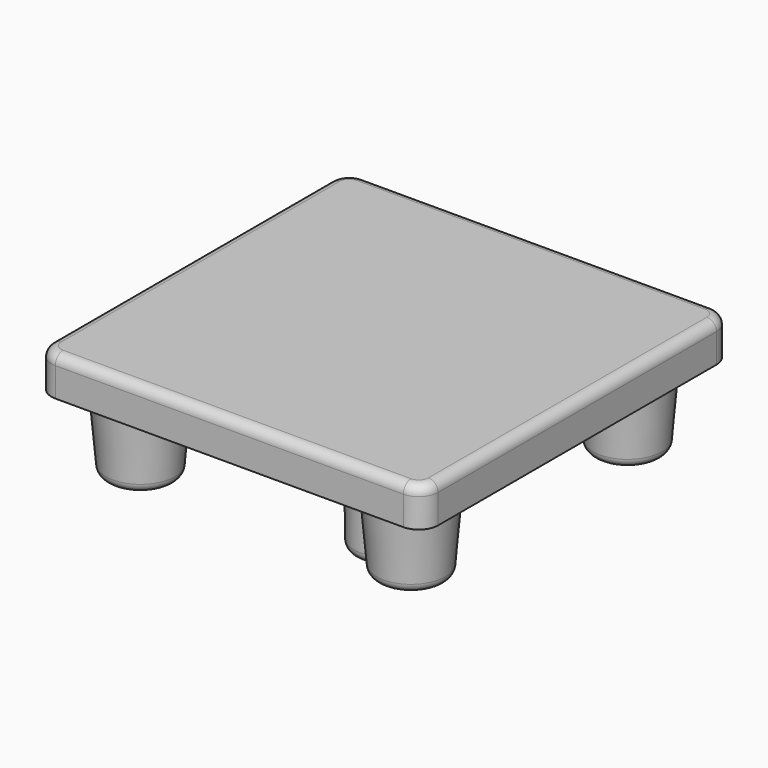
from build123d import *

# Parameters (mm, degrees)
F0_W                     = 20
F0_H                     = 20
F0_R                     = 2.1
F1_DEPTH                 = 2
F2_DEPTH                 = 4
F2_TAPER                 = 5
F3_DEPTH                 = 8
DRAFT_F3_DRAFTED_ANGLE   = 1
DRAFT_F3_2_DRAFTED_ANGLE = 1
F4_R                     = 1
F5_T12_ANGLE             = 249.4018409202
F5_T17_ANGLE             = 249.4018409202
F5_T19_DEPTH             = 18
F5_T21_DEPTH             = 18
F5_T24_ANGLE             = 90
F5_T26_ANGLE             = 90
F5_T28_ANGLE             = 90
F5_T30_ANGLE             = 90
F5_T42_ANGLE             = 245.17376067
F5_T47_ANGLE             = 245.17376067


# Not quite as in the source:
# - a fillet or chamfer that OpenCascade refuses, or shapes differently, is made with other operations: its cross-section is extruded or revolved along the edge and cut away or added
# - an extrude with a draft is written as a straight extrude whose walls are then drafted


with BuildPart() as f1:
    # F0 (on Top) → F1 (new body)
    with BuildSketch(Plane.XY):
        with Locations((-49.5571177453, 39.7264205217)):
            Rectangle(F0_W, F0_H)
        with Locations((-56.5571177453, 32.7264205217)):
            Circle(F0_R, mode=Mode.SUBTRACT)
        with BuildLine():
            ThreePointArc((-47.8689234437, 39.9264205217), (-47.8600717364, 39.8265945884), (-47.8571177453, 39.7264205217))
            ThreePointArc((-47.8571177453, 39.7264205217), (-47.8600717364, 39.6262464551), (-47.8689234437, 39.5264205217))
            ThreePointArc((-47.8689234437, 39.5264205217), (-49.5571177453, 38.0264205217), (-51.2453120469, 39.5264205217))
            ThreePointArc((-51.2453120469, 39.5264205217), (-51.2571177453, 39.7264205217), (-51.2453120469, 39.9264205217))
            ThreePointArc((-51.2453120469, 39.9264205217), (-49.5571177453, 41.4264205217), (-47.8689234437, 39.9264205217))
        make_face(mode=Mode.SUBTRACT)
        with Locations((-42.5571177453, 32.7264205217)):
            Circle(F0_R, mode=Mode.SUBTRACT)
        with Locations((-56.5571177453, 46.7264205217)):
            Circle(F0_R, mode=Mode.SUBTRACT)
        with Locations((-42.5571177453, 46.7264205217)):
            Circle(F0_R, mode=Mode.SUBTRACT)
        with Locations((-42.5571177453, 46.7264205217)):
            Circle(F0_R)
        with Locations((-42.5571177453, 32.7264205217)):
            Circle(F0_R)
        with Locations((-56.5571177453, 32.7264205217)):
            Circle(F0_R)
        with Locations((-56.5571177453, 46.7264205217)):
            Circle(F0_R)
        with BuildLine():
            ThreePointArc((-47.8689234437, 39.5264205217), (-47.8600717364, 39.6262464551), (-47.8571177453, 39.7264205217))
            ThreePointArc((-47.8571177453, 39.7264205217), (-47.8600717364, 39.8265945884), (-47.8689234437, 39.9264205217))
            Line((-47.8689234437, 39.9264205217), (-51.2453120469, 39.9264205217))
            ThreePointArc((-51.2453120469, 39.9264205217), (-51.2571177453, 39.7264205217), (-51.2453120469, 39.5264205217))
            Line((-51.2453120469, 39.5264205217), (-47.8689234437, 39.5264205217))
        make_face()
        with BuildLine():
            Line((-51.2453120469, 39.9264205217), (-47.8689234437, 39.9264205217))
            ThreePointArc((-47.8689234437, 39.9264205217), (-49.5571177453, 41.4264205217), (-51.2453120469, 39.9264205217))
        make_face()
        with BuildLine():
            ThreePointArc((-51.2453120469, 39.5264205217), (-49.5571177453, 38.0264205217), (-47.8689234437, 39.5264205217))
            Line((-47.8689234437, 39.5264205217), (-51.2453120469, 39.5264205217))
        make_face()
    extrude(amount=F1_DEPTH)

    # F0 (on Top) → F2 (join)
    with BuildSketch(Plane.XY):
        with Locations((-42.5571177453, 46.7264205217)):
            Circle(F0_R)
        with Locations((-56.5571177453, 46.7264205217)):
            Circle(F0_R)
        with Locations((-56.5571177453, 32.7264205217)):
            Circle(F0_R)
        with Locations((-42.5571177453, 32.7264205217)):
            Circle(F0_R)
    extrude(amount=-F2_DEPTH, taper=F2_TAPER)


with BuildPart() as f3_drafted:
    # F0 (on Top) → F3 (new body)
    with BuildSketch(Plane.XY):
        with BuildLine():
            Line((-51.2453120469, 39.9264205217), (-47.8689234437, 39.9264205217))
            ThreePointArc((-47.8689234437, 39.9264205217), (-49.5571177453, 41.4264205217), (-51.2453120469, 39.9264205217))
        make_face()
    extrude(amount=-F3_DEPTH)

    # draft_F3_drafted
    draft_f3_drafted_walls = [f3_drafted.faces().sort_by_distance(p)[0] for p in [
        (-49.5571177453, 39.9264205217, -5.3333333333),
        (-49.5571177453, 41.4264205217, -5.3333333333),
    ]]
    draft(draft_f3_drafted_walls, neutral_plane=Plane(origin=(0, 0, 0), x_dir=(1, 0, 0), z_dir=(0, 0, -1)), angle=DRAFT_F3_DRAFTED_ANGLE)


with BuildPart() as f1_1:
    add(f1.part)

    # join_F3_drafted: union F3_drafted
    add(f3_drafted.part)


with BuildPart() as f3_2_drafted:
    # F0 (on Top) → F3, piece 2 (new body)
    with BuildSketch(Plane.XY):
        with BuildLine():
            ThreePointArc((-51.2453120469, 39.5264205217), (-49.5571177453, 38.0264205217), (-47.8689234437, 39.5264205217))
            Line((-47.8689234437, 39.5264205217), (-51.2453120469, 39.5264205217))
        make_face()
    extrude(amount=-F3_DEPTH)

    # draft_F3_2_drafted
    draft_f3_2_drafted_walls = [f3_2_drafted.faces().sort_by_distance(p)[0] for p in [
        (-49.5571177453, 38.0264205217, -5.3333333333),
        (-49.5571177453, 39.5264205217, -5.3333333333),
    ]]
    draft(draft_f3_2_drafted_walls, neutral_plane=Plane(origin=(0, 0, 0), x_dir=(1, 0, 0), z_dir=(0, 0, -1)), angle=DRAFT_F3_2_DRAFTED_ANGLE)


with BuildPart() as f1_2:
    add(f1_1.part)

    # join_F3_2_drafted: union F3_2_drafted
    add(f3_2_drafted.part)

    # F4
    f4_edges = [f1_2.edges().sort_by_distance(p)[0] for p in [
        (-39.557118, 49.726421, 1),
        (-39.557118, 29.726421, 1),
        (-59.557118, 49.726421, 1),
        (-59.557118, 29.726421, 1),
    ]]
    fillet(f4_edges, radius=F4_R)

    # F5: fillet of radius 0.5 on 20 edges, made by hand

    # F5_s1 → F5_t2 (revolve)
    with BuildSketch(Plane.XZ.offset(-46.7264205217)):
        with BuildLine():
            ThreePointArc((-39.9989521583, 0), (-40.3367472621, -0.1313613316), (-40.4970495073, -0.4564221286))
            Line((-40.4970495073, -0.4564221286), (-40.5070114543, -0.4555505712))
            Line((-40.5070114543, -0.4555505712), (-40.466281057, 0.01))
            Line((-40.466281057, 0.01), (-39.9989521583, 0.01))
            Line((-39.9989521583, 0.01), (-39.9989521583, 0))
        make_face()
    revolve(axis=Axis((-42.5571177453, 46.7264205217, 0), (0, 0, -1)))

    # F5_s3 → F5_t4 (revolve)
    with BuildSketch(Plane.XZ.offset(-32.7264205217)):
        with BuildLine():
            ThreePointArc((-39.9989521583, 0), (-40.3367472621, -0.1313613316), (-40.4970495073, -0.4564221286))
            Line((-40.4970495073, -0.4564221286), (-40.5070114543, -0.4555505712))
            Line((-40.5070114543, -0.4555505712), (-40.466281057, 0.01))
            Line((-40.466281057, 0.01), (-39.9989521583, 0.01))
            Line((-39.9989521583, 0.01), (-39.9989521583, 0))
        make_face()
    revolve(axis=Axis((-42.5571177453, 32.7264205217, 0), (0, 0, -1)))

    # F5_s5 → F5_t6 (revolve)
    with BuildSketch(Plane.XZ.offset(-32.7264205217)):
        with BuildLine():
            ThreePointArc((-53.9989521583, 0), (-54.3367472621, -0.1313613316), (-54.4970495073, -0.4564221286))
            Line((-54.4970495073, -0.4564221286), (-54.5070114543, -0.4555505712))
            Line((-54.5070114543, -0.4555505712), (-54.466281057, 0.01))
            Line((-54.466281057, 0.01), (-53.9989521583, 0.01))
            Line((-53.9989521583, 0.01), (-53.9989521583, 0))
        make_face()
    revolve(axis=Axis((-56.5571177453, 32.7264205217, 0), (0, 0, -1)))

    # F5_s7 → F5_t8 (revolve)
    with BuildSketch(Plane.XZ.offset(-46.7264205217)):
        with BuildLine():
            ThreePointArc((-53.9989521583, 0), (-54.3367472621, -0.1313613316), (-54.4970495073, -0.4564221286))
            Line((-54.4970495073, -0.4564221286), (-54.5070114543, -0.4555505712))
            Line((-54.5070114543, -0.4555505712), (-54.466281057, 0.01))
            Line((-54.466281057, 0.01), (-53.9989521583, 0.01))
            Line((-53.9989521583, 0.01), (-53.9989521583, 0))
        make_face()
    revolve(axis=Axis((-56.5571177453, 46.7264205217, 0), (0, 0, -1)))


with BuildPart() as f5_tool10:
    # F5_s11 → F5_t12 (revolve)
    with BuildSketch(Plane(origin=(2.5321968025, 3.6568310809, 0), x_dir=(0, 0, 1), z_dir=(0.5692927311, 0.8221348954, 0))):
        with BuildLine():
            ThreePointArc((0, -65.5499468838), (-0.1433747754, -65.1994922516), (-0.4912737968, -65.0500230362))
            Line((-0.4912737968, -65.0500230362), (-0.4910992727, -65.0400245593))
            Line((-0.4910992727, -65.0400245593), (0.01, -65.0487712796))
            Line((0.01, -65.0487712796), (0.01, -65.5499468838))
            Line((0.01, -65.5499468838), (0, -65.5499468838))
        make_face()
    revolve(axis=Axis((-49.5571177453, 39.7264205217, 0), (0, 0, 1)), revolution_arc=F5_T12_ANGLE)

    split(bisect_by=Plane(origin=(0, 39.514381308, -0.6897260913), x_dir=(1, 0, 0), z_dir=(0, -0.9998476952, 0.0174524064)), keep=Keep.TOP)


with BuildPart() as f1_3:
    add(f1_2.part)

    # F5_t9: union F5_tool10
    add(f5_tool10.part)


with BuildPart() as f5_tool15:
    # F5_s16 → F5_t17 (revolve)
    with BuildSketch(Plane(origin=(2.5321968025, 3.6568310809, 0), x_dir=(0, 0, 1), z_dir=(-0.5692927311, -0.8221348954, 0))):
        with BuildLine():
            ThreePointArc((0, 61.1672496207), (-0.1433747754, 61.5177042528), (-0.4912737968, 61.6671734683))
            Line((-0.4912737968, 61.6671734683), (-0.4910992727, 61.6771719452))
            Line((-0.4910992727, 61.6771719452), (0.01, 61.6684252249))
            Line((0.01, 61.6684252249), (0.01, 61.1672496207))
            Line((0.01, 61.1672496207), (0, 61.1672496207))
        make_face()
    revolve(axis=Axis((-49.5571177453, 39.7264205217, 0), (0, 0, 1)), revolution_arc=F5_T17_ANGLE)

    split(bisect_by=Plane(origin=(0, 39.9142594734, 0.6967059907), x_dir=(1, 0, 0), z_dir=(0, 0.9998476952, 0.0174524064)), keep=Keep.TOP)


with BuildPart() as f1_4:
    add(f1_3.part)

    # F5_t14: union F5_tool15
    add(f5_tool15.part)

    # F5_s20 → F5_t19 (cut)
    with BuildSketch(Plane.YZ.offset(-58.5571177453)):
        with BuildLine():
            ThreePointArc((49.7264205217, 1.5), (49.5799739123, 1.8535533906), (49.2264205217, 2))
            Line((49.2264205217, 2), (49.2264205217, 2.01))
            Line((49.2264205217, 2.01), (49.7364205217, 2.01))
            Line((49.7364205217, 2.01), (49.7364205217, 1.5))
            Line((49.7364205217, 1.5), (49.7264205217, 1.5))
        make_face()
        with BuildLine():
            ThreePointArc((30.2264205217, 2), (29.8728671311, 1.8535533906), (29.7264205217, 1.5))
            Line((29.7264205217, 1.5), (29.7164205217, 1.5))
            Line((29.7164205217, 1.5), (29.7164205217, 2.01))
            Line((29.7164205217, 2.01), (30.2264205217, 2.01))
            Line((30.2264205217, 2.01), (30.2264205217, 2))
        make_face()
    extrude(amount=F5_T19_DEPTH, mode=Mode.SUBTRACT)

    # F5_s22 → F5_t21 (cut)
    with BuildSketch(Plane.XZ.offset(-48.7264205217)):
        with BuildLine():
            ThreePointArc((-40.0571177453, 2), (-39.7035643547, 1.8535533906), (-39.5571177453, 1.5))
            Line((-39.5571177453, 1.5), (-39.5471177453, 1.5))
            Line((-39.5471177453, 1.5), (-39.5471177453, 2.01))
            Line((-39.5471177453, 2.01), (-40.0571177453, 2.01))
            Line((-40.0571177453, 2.01), (-40.0571177453, 2))
        make_face()
        with BuildLine():
            ThreePointArc((-59.0571177453, 2), (-59.4106711359, 1.8535533906), (-59.5571177453, 1.5))
            Line((-59.5571177453, 1.5), (-59.5671177453, 1.5))
            Line((-59.5671177453, 1.5), (-59.5671177453, 2.01))
            Line((-59.5671177453, 2.01), (-59.0571177453, 2.01))
            Line((-59.0571177453, 2.01), (-59.0571177453, 2))
        make_face()
    extrude(amount=F5_T21_DEPTH, mode=Mode.SUBTRACT)

    # F5_s23 → F5_t24 (revolve, cut)
    with BuildSketch(Plane.YZ.offset(-40.5571177453)):
        with BuildLine():
            ThreePointArc((49.2264205217, 2), (49.5799739123, 1.8535533906), (49.7264205217, 1.5))
            Line((49.7264205217, 1.5), (49.7364205217, 1.5))
            Line((49.7364205217, 1.5), (49.7364205217, 2.01))
            Line((49.7364205217, 2.01), (49.2264205217, 2.01))
            Line((49.2264205217, 2.01), (49.2264205217, 2))
        make_face()
    revolve(axis=Axis((-40.5571177453, 48.7264205217, 2), (0, 0, -1)), revolution_arc=F5_T24_ANGLE, mode=Mode.SUBTRACT)

    # F5_s25 → F5_t26 (revolve, cut)
    with BuildSketch(Plane.YZ.offset(-58.5571177453)):
        with BuildLine():
            ThreePointArc((49.2264205217, 2), (49.5799739123, 1.8535533906), (49.7264205217, 1.5))
            Line((49.7264205217, 1.5), (49.7364205217, 1.5))
            Line((49.7364205217, 1.5), (49.7364205217, 2.01))
            Line((49.7364205217, 2.01), (49.2264205217, 2.01))
            Line((49.2264205217, 2.01), (49.2264205217, 2))
        make_face()
    revolve(axis=Axis((-58.5571177453, 48.7264205217, 2), (0, 0, 1)), revolution_arc=F5_T26_ANGLE, mode=Mode.SUBTRACT)

    # F5_s27 → F5_t28 (revolve, cut)
    with BuildSketch(Plane.XZ.offset(-30.7264205217)):
        with BuildLine():
            ThreePointArc((-40.0571177453, 2), (-39.7035643547, 1.8535533906), (-39.5571177453, 1.5))
            Line((-39.5571177453, 1.5), (-39.5471177453, 1.5))
            Line((-39.5471177453, 1.5), (-39.5471177453, 2.01))
            Line((-39.5471177453, 2.01), (-40.0571177453, 2.01))
            Line((-40.0571177453, 2.01), (-40.0571177453, 2))
        make_face()
    revolve(axis=Axis((-40.5571177453, 30.7264205217, 2), (0, 0, -1)), revolution_arc=F5_T28_ANGLE, mode=Mode.SUBTRACT)

    # F5_s29 → F5_t30 (revolve, cut)
    with BuildSketch(Plane.XZ.offset(-30.7264205217)):
        with BuildLine():
            ThreePointArc((-59.0571177453, 2), (-59.4106711359, 1.8535533906), (-59.5571177453, 1.5))
            Line((-59.5571177453, 1.5), (-59.5671177453, 1.5))
            Line((-59.5671177453, 1.5), (-59.5671177453, 2.01))
            Line((-59.5671177453, 2.01), (-59.0571177453, 2.01))
            Line((-59.0571177453, 2.01), (-59.0571177453, 2))
        make_face()
    revolve(axis=Axis((-58.5571177453, 30.7264205217, 2), (0, 0, 1)), revolution_arc=F5_T30_ANGLE, mode=Mode.SUBTRACT)

    # F5_s31 → F5_t32 (revolve, cut)
    with BuildSketch(Plane.XZ.offset(-46.7264205217)):
        with BuildLine():
            ThreePointArc((-40.7671406373, -3.5435778714), (-40.9274428826, -3.8686386684), (-41.2652379864, -4))
            Line((-41.2652379864, -4), (-41.2652379864, -4.01))
            Line((-41.2652379864, -4.01), (-40.7979090876, -4.01))
            Line((-40.7979090876, -4.01), (-40.7571786904, -3.5444494288))
            Line((-40.7571786904, -3.5444494288), (-40.7671406373, -3.5435778714))
        make_face()
    revolve(axis=Axis((-42.5571177453, 46.7264205217, -4), (0, 0, 1)), mode=Mode.SUBTRACT)

    # F5_s33 → F5_t34 (revolve, cut)
    with BuildSketch(Plane.XZ.offset(-46.7264205217)):
        with BuildLine():
            ThreePointArc((-54.7671406373, -3.5435778714), (-54.9274428826, -3.8686386684), (-55.2652379864, -4))
            Line((-55.2652379864, -4), (-55.2652379864, -4.01))
            Line((-55.2652379864, -4.01), (-54.7979090876, -4.01))
            Line((-54.7979090876, -4.01), (-54.7571786904, -3.5444494288))
            Line((-54.7571786904, -3.5444494288), (-54.7671406373, -3.5435778714))
        make_face()
    revolve(axis=Axis((-56.5571177453, 46.7264205217, -4), (0, 0, 1)), mode=Mode.SUBTRACT)

    # F5_s35 → F5_t36 (revolve, cut)
    with BuildSketch(Plane.XZ.offset(-32.7264205217)):
        with BuildLine():
            ThreePointArc((-54.7671406373, -3.5435778714), (-54.9274428826, -3.8686386684), (-55.2652379864, -4))
            Line((-55.2652379864, -4), (-55.2652379864, -4.01))
            Line((-55.2652379864, -4.01), (-54.7979090876, -4.01))
            Line((-54.7979090876, -4.01), (-54.7571786904, -3.5444494288))
            Line((-54.7571786904, -3.5444494288), (-54.7671406373, -3.5435778714))
        make_face()
    revolve(axis=Axis((-56.5571177453, 32.7264205217, -4), (0, 0, 1)), mode=Mode.SUBTRACT)

    # F5_s37 → F5_t38 (revolve, cut)
    with BuildSketch(Plane.XZ.offset(-32.7264205217)):
        with BuildLine():
            ThreePointArc((-40.7671406373, -3.5435778714), (-40.9274428826, -3.8686386684), (-41.2652379864, -4))
            Line((-41.2652379864, -4), (-41.2652379864, -4.01))
            Line((-41.2652379864, -4.01), (-40.7979090876, -4.01))
            Line((-40.7979090876, -4.01), (-40.7571786904, -3.5444494288))
            Line((-40.7571786904, -3.5444494288), (-40.7671406373, -3.5435778714))
        make_face()
    revolve(axis=Axis((-42.5571177453, 32.7264205217, -4), (0, 0, 1)), mode=Mode.SUBTRACT)


with BuildPart() as f5_tool40:
    # F5_s41 → F5_t42 (revolve)
    with BuildSketch(Plane(origin=(3.6527167463, 5.7144764534, 0), x_dir=(0, 0, 1), z_dir=(0.538577865, 0.8425757434, 0))):
        with BuildLine():
            ThreePointArc((-8, -64.2204069217), (-7.8566252246, -64.5708615538), (-7.5087262032, -64.7203307692))
            Line((-7.5087262032, -64.7203307692), (-7.5089007273, -64.7303292462))
            Line((-7.5089007273, -64.7303292462), (-8.01, -64.7215825258))
            Line((-8.01, -64.7215825258), (-8.01, -64.2204069217))
            Line((-8.01, -64.2204069217), (-8, -64.2204069217))
        make_face()
    revolve(axis=Axis((-49.5571177453, 39.7264205217, -8), (0, 0, 1)), revolution_arc=F5_T42_ANGLE)

    split(bisect_by=Plane(origin=(0, 39.514381308, -0.6897260913), x_dir=(1, 0, 0), z_dir=(0, -0.9998476952, 0.0174524064)), keep=Keep.TOP)


with BuildPart() as f1_5:
    add(f1_4.part)

    # F5_t39: cut F5_tool40
    add(f5_tool40.part, mode=Mode.SUBTRACT)


with BuildPart() as f5_tool45:
    # F5_s46 → F5_t47 (revolve)
    with BuildSketch(Plane(origin=(3.6527167463, 5.7144764534, 0), x_dir=(0, 0, 1), z_dir=(-0.538577865, -0.8425757434, 0))):
        with BuildLine():
            ThreePointArc((-8, 62.0823852236), (-7.8566252246, 61.7319305915), (-7.5087262032, 61.582461376))
            Line((-7.5087262032, 61.582461376), (-7.5089007273, 61.5724628991))
            Line((-7.5089007273, 61.5724628991), (-8.01, 61.5812096194))
            Line((-8.01, 61.5812096194), (-8.01, 62.0823852236))
            Line((-8.01, 62.0823852236), (-8, 62.0823852236))
        make_face()
    revolve(axis=Axis((-49.5571177453, 39.7264205217, -8), (0, 0, 1)), revolution_arc=F5_T47_ANGLE)

    split(bisect_by=Plane(origin=(0, 39.9142594734, 0.6967059907), x_dir=(1, 0, 0), z_dir=(0, 0.9998476952, 0.0174524064)), keep=Keep.TOP)


with BuildPart() as f1_6:
    add(f1_5.part)

    # F5_t44: cut F5_tool45
    add(f5_tool45.part, mode=Mode.SUBTRACT)


solid = f1_6.part
